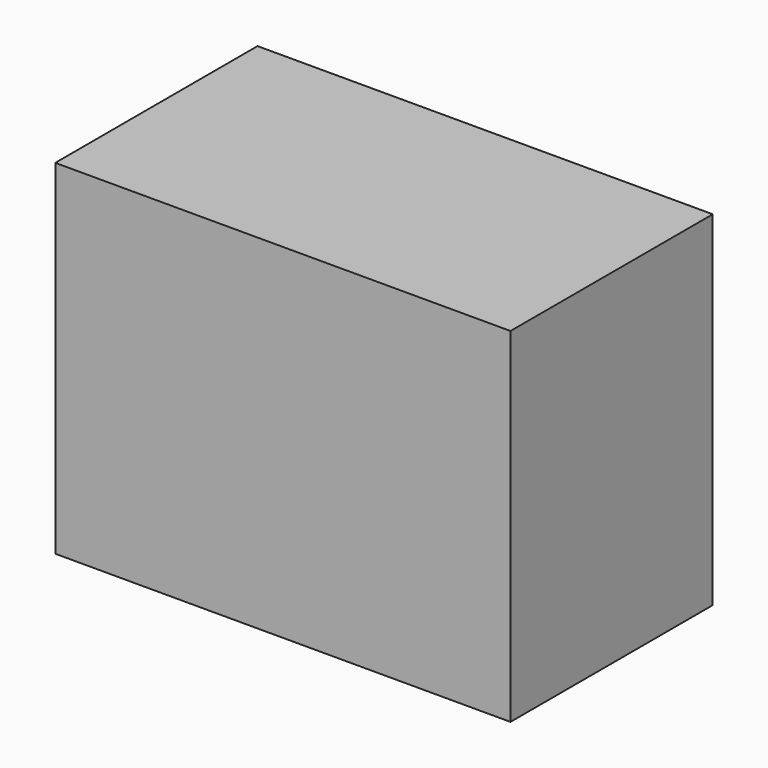
from build123d import *

# Parameters (mm, degrees)
F0_W     = 224.0990400314
F0_H     = 169.4250032306
F1_DEPTH = 124.46


# Not quite as in the source:
# - the program builds the solid bodies; features that only make, move or delete a surface that nothing else refers to are left out


with BuildPart() as f1:
    # F0 (on Front) → F1 (new body)
    with BuildSketch(Plane.XZ):
        with Locations((-37.5905483961, 10.0628472865)):
            Rectangle(F0_W, F0_H)
    extrude(amount=-F1_DEPTH)


solid = f1.part
